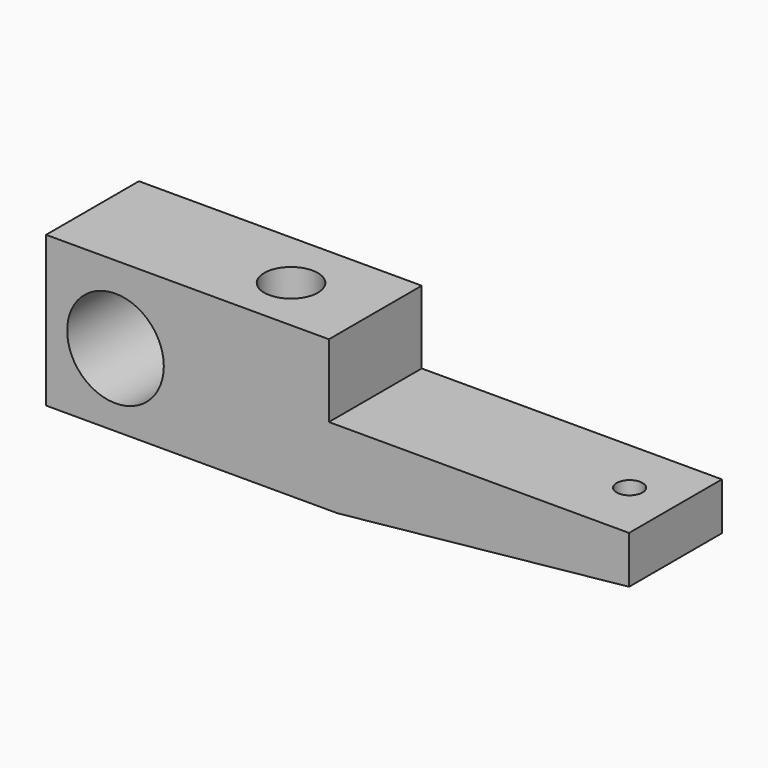
from build123d import *

# Parameters (mm, degrees)
F0_R     = 10.5768156475
F1_DEPTH = 25.4
F2_R     = 5.8673814398
F3_DEPTH = 32.9165069776
F5_R     = 2.8308188493
F6_DEPTH = 16.9651473331


# Not quite as in the source:
# - a feature names something its author has since deleted; it is built from what else it names


with BuildPart() as f1:
    # F0 (on Front) → F1 (new body)
    with BuildSketch(Plane.XZ):
        Polygon((0, 38.612421602), (-61.9064718485, 38.612421602), (-61.9064718485, 5.6969146244), (1.8989704549, 5.6969146244), (65.7044127584, 12.2800152749), (65.7044127584, 22.1546681132), (65.7044127584, 22.6610619575), (0, 22.6610619575), align=None)
        with Locations((-46.7147007585, 21.6482765973)):
            Circle(F0_R, mode=Mode.SUBTRACT)
    extrude(amount=F1_DEPTH)

    # F2 (on face) → F3 (cut, through all)
    with BuildSketch(Plane.XY.offset(38.612421602)):
        with Locations((-18.1035287678, -13.1292007864)):
            Circle(F2_R)
    extrude(amount=-F3_DEPTH, mode=Mode.SUBTRACT)

    # F5 (on face) → F6 (cut, through all)
    with BuildSketch(Plane.XY.offset(22.6610619575)):
        with Locations((55.3233735263, -12.2800152749)):
            Circle(F5_R)
    extrude(amount=-F6_DEPTH, mode=Mode.SUBTRACT)


solid = f1.part
